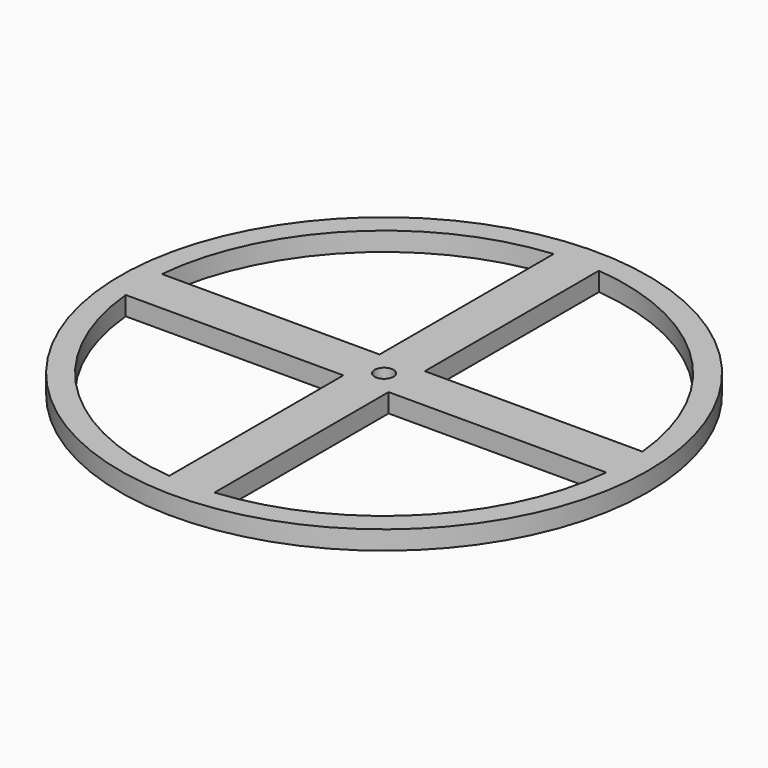
from build123d import *

# Parameters (mm, degrees)
F0_R     = 44.45
F0_R_2   = 1.5875
F1_DEPTH = 3.175


# Not quite as in the source:
# - a length typed as a fraction of an inch, garbled in the dataset ("3 / 203.2 mm" for 3/8 in), is restored


with BuildPart() as f1:
    # F0 (on Top) → F1 (new body)
    with BuildSketch(Plane.XY):
        Circle(F0_R)
        with BuildLine():
            ThreePointArc((40.4610120981, 3.81), (40.5952283629, 1.9071009851), (40.64, 0))
            ThreePointArc((40.64, 0), (40.5952283629, -1.9071009851), (40.4610120981, -3.81))
            ThreePointArc((40.4610120981, -3.81), (28.7368195874, -28.7368195874), (3.81, -40.4610120981))
            ThreePointArc((3.81, -40.4610120981), (0, -40.64), (-3.81, -40.4610120981))
            ThreePointArc((-3.81, -40.4610120981), (-28.7368195874, -28.7368195874), (-40.4610120981, -3.81))
            ThreePointArc((-40.4610120981, -3.81), (-40.64, 0), (-40.4610120981, 3.81))
            ThreePointArc((-40.4610120981, 3.81), (-28.7368195874, 28.7368195874), (-3.81, 40.4610120981))
            ThreePointArc((-3.81, 40.4610120981), (0, 40.64), (3.81, 40.4610120981))
            ThreePointArc((3.81, 40.4610120981), (28.7368195874, 28.7368195874), (40.4610120981, 3.81))
        make_face(mode=Mode.SUBTRACT)
        with BuildLine():
            ThreePointArc((40.4610120981, -3.81), (40.5952283629, -1.9071009851), (40.64, 0))
            ThreePointArc((40.64, 0), (40.5952283629, 1.9071009851), (40.4610120981, 3.81))
            Line((40.4610120981, 3.81), (3.81, 3.81))
            Line((3.81, 3.81), (3.81, 0))
            Line((3.81, 0), (3.81, -3.81))
            Line((3.81, -3.81), (40.4610120981, -3.81))
        make_face()
        with BuildLine():
            Line((3.81, 3.81), (3.81, 40.4610120981))
            ThreePointArc((3.81, 40.4610120981), (0, 40.64), (-3.81, 40.4610120981))
            Line((-3.81, 40.4610120981), (-3.81, 3.81))
            Line((-3.81, 3.81), (0, 3.81))
            Line((0, 3.81), (3.81, 3.81))
        make_face()
        Polygon((3.81, 0), (3.81, 3.81), (0, 3.81), (-3.81, 3.81), (-3.81, 0), (-3.81, -3.81), (0, -3.81), (3.81, -3.81), align=None)
        Circle(F0_R_2, mode=Mode.SUBTRACT)
        with BuildLine():
            ThreePointArc((-3.81, -40.4610120981), (0, -40.64), (3.81, -40.4610120981))
            Line((3.81, -40.4610120981), (3.81, -3.81))
            Line((3.81, -3.81), (0, -3.81))
            Line((0, -3.81), (-3.81, -3.81))
            Line((-3.81, -3.81), (-3.81, -40.4610120981))
        make_face()
        with BuildLine():
            Line((-3.81, 3.81), (-40.4610120981, 3.81))
            ThreePointArc((-40.4610120981, 3.81), (-40.64, 0), (-40.4610120981, -3.81))
            Line((-40.4610120981, -3.81), (-3.81, -3.81))
            Line((-3.81, -3.81), (-3.81, 0))
            Line((-3.81, 0), (-3.81, 3.81))
        make_face()
    extrude(amount=F1_DEPTH)


solid = f1.part
